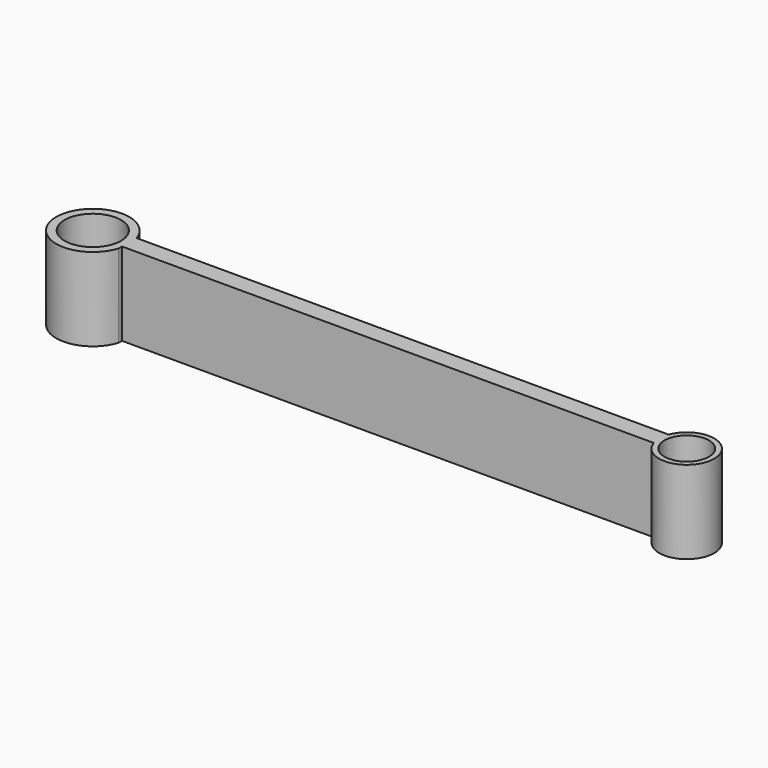
from build123d import *

# Parameters (mm, degrees)
F0_R     = 8.5
F0_R_2   = 6.6901913145
F1_DEPTH = 25


# Not quite as in the source:
# - a feature names something its author has since deleted; it is built from what else it names


with BuildPart() as f1:
    # F0 (on Top) → F1 (new body)
    with BuildSketch(Plane.XY):
        with BuildLine():
            Line((147.8986507368, 41.0247598798), (-12.1013492632, 41.0247598798))
            ThreePointArc((-12.1013492632, 41.0247598798), (-33.5643369753, 37.6297800364), (-12.1013492632, 34.2348001929))
            Line((-12.1013492632, 34.2348001929), (-12.1013492632, 35.5247598798))
            Line((-12.1013492632, 35.5247598798), (147.8986507368, 35.5247598798))
            ThreePointArc((147.8986507368, 35.5247598798), (164.0425617184, 38.1300025139), (147.8986507368, 40.735245148))
            Line((147.8986507368, 40.735245148), (147.8986507368, 41.0247598798))
        make_face()
        with Locations((-22.5643369753, 37.6297800364)):
            Circle(F0_R, mode=Mode.SUBTRACT)
        with Locations((155.7603941795, 38.1300025139)):
            Circle(F0_R_2, mode=Mode.SUBTRACT)
    extrude(amount=F1_DEPTH)


solid = f1.part
